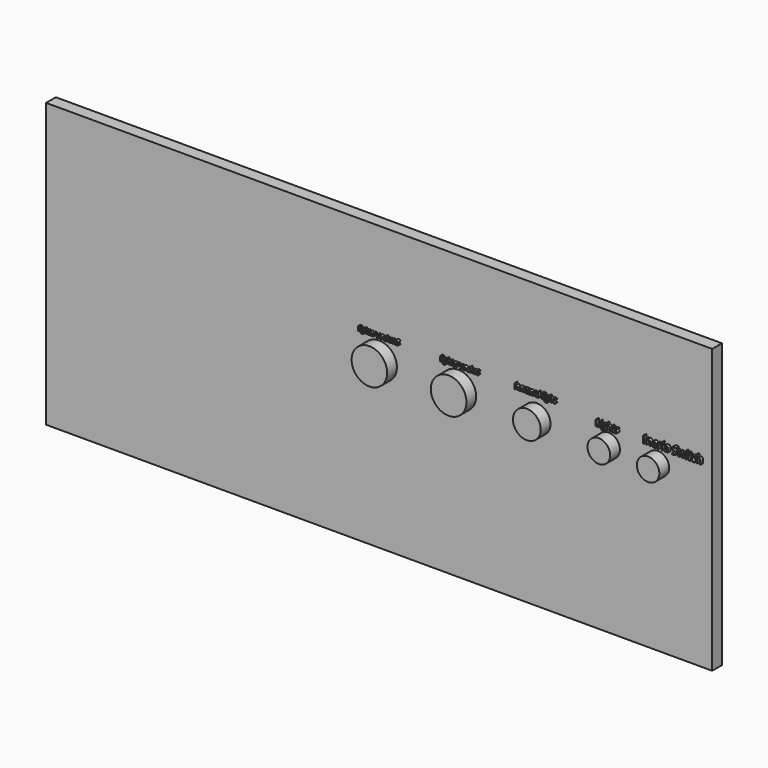
from build123d import *

# Parameters (mm, degrees)
F0_W           = 208.1463187933
F0_H           = 88.5524228215
F1_DEPTH       = 3.81
F2_R           = 3.5481005897
F2_R_2         = 4.3403151598
F2_R_3         = 5.5629550831
F2_R_4         = 5.5528690672
F2_R_5         = 3.5146674086
F3_DEPTH       = 3.81
F4_TEXT_SIZE   = 2.1720592155
F4_TEXT_SIZE_2 = 1.939070067
F4_TEXT_SIZE_3 = 1.7916106421
F4_TEXT_SIZE_4 = 2.5404668931
F4_TEXT_SIZE_5 = 3.1017336167
F5_DEPTH       = 1.016


# Not quite as in the source:
# - Text() gives the source's letters only with a copy of the font that has no kerning and outlines rounded to 1/6400 em; it was checked with that copy


with BuildPart() as f1:
    # F0 (on Front) → F1 (new body)
    with BuildSketch(Plane.XZ):
        Rectangle(F0_W, F0_H)
    extrude(amount=F1_DEPTH)

    # F2 (on face) → F3 (join)
    with BuildSketch(Plane.XZ.offset(3.81)):
        with Locations((71.7059746385, 7.1895709261)):
            Circle(F2_R)
        with Locations((49.2158867419, 7.1895709261)):
            Circle(F2_R_2)
        with Locations((24.7645713389, 7.1895709261)):
            Circle(F2_R_3)
        with Locations((0, 7.1895709261)):
            Circle(F2_R_4)
        with Locations((87.1009379625, 7.1895709261)):
            Circle(F2_R_5)
    extrude(amount=F3_DEPTH)

    # F4 (on face) → F5 (join)
    with BuildSketch(Plane.XZ.offset(3.81)):
        with Locations((42.8984212004, 13.7859994559)):
            Text('harzard light', F4_TEXT_SIZE, font='Open Sans', text_align=(TextAlign.LEFT, TextAlign.BOTTOM))
        with Locations((19.6053911392, 13.8240124527)):
            Text('lighter socket', F4_TEXT_SIZE_2, font='Open Sans', text_align=(TextAlign.LEFT, TextAlign.BOTTOM))
        with Locations((-5.9183216654, 13.8801330322)):
            Text('lighter socket 2', F4_TEXT_SIZE_3, font='Open Sans', text_align=(TextAlign.LEFT, TextAlign.BOTTOM))
        with Locations((68.2329162955, 11.8593191728)):
            Text('Lights', F4_TEXT_SIZE_4, font='Open Sans', text_align=(TextAlign.LEFT, TextAlign.BOTTOM))
        with Locations((83.0172821879, 11.8873277679)):
            Text('Ineria Switch', F4_TEXT_SIZE_5, font='Open Sans', text_align=(TextAlign.LEFT, TextAlign.BOTTOM))
    extrude(amount=F5_DEPTH)


solid = f1.part
